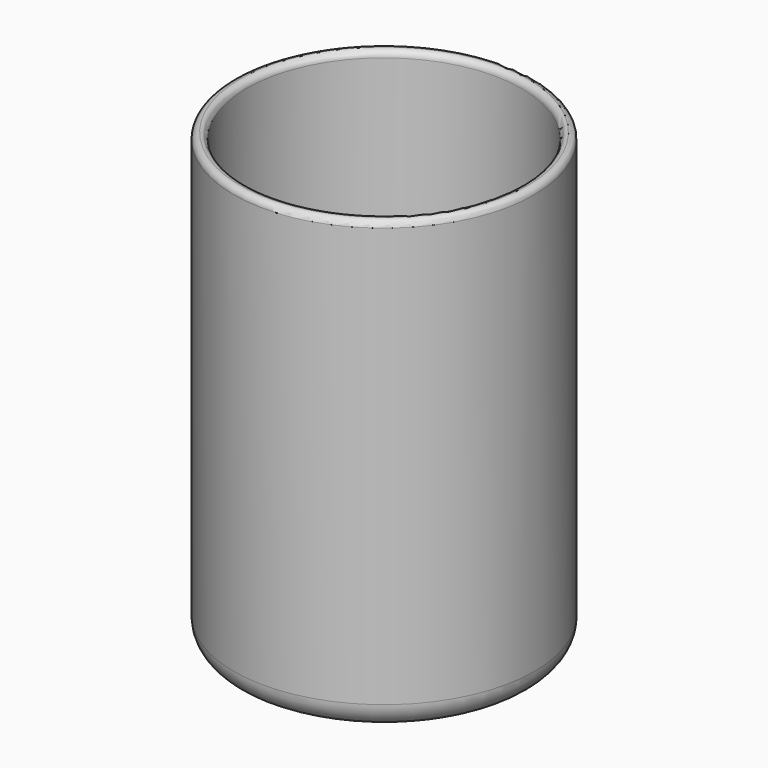
from build123d import *

# Parameters (mm, degrees)
F0_R     = 30
F1_DEPTH = 90
F2_T     = -2.5
F3_R     = 2.5
F4_R     = 5
F5_R     = 1.24999


# Not quite as in the source:
# - a fillet or chamfer is up to 0.001 mm smaller than in the source, because OpenCascade refuses the exact size


with BuildPart() as f1:
    # F0 (on Top) → F1 (new body)
    with BuildSketch(Plane.XY):
        Circle(F0_R)
    extrude(amount=F1_DEPTH)

    # F2
    f2_openings = [f1.faces().sort_by_distance(p)[0] for p in [
        (0, 0, 90),
    ]]
    offset(amount=F2_T, openings=f2_openings)

    # F3
    f3_edges = [f1.edges().sort_by_distance(p)[0] for p in [
        (-27.5, 0, 2.5),
    ]]
    fillet(f3_edges, radius=F3_R)

    # F4
    f4_edges = [f1.edges().sort_by_distance(p)[0] for p in [
        (-30, 0, 0),
    ]]
    fillet(f4_edges, radius=F4_R)

    # F5 (radius 1.25 in the source; OpenCascade refuses exactly that, so slightly less here)
    f5_edges = [f1.edges().sort_by_distance(p)[0] for p in [
        (-30, 0, 90),
        (-27.5, 0, 90),
    ]]
    fillet(f5_edges, radius=F5_R)


solid = f1.part
